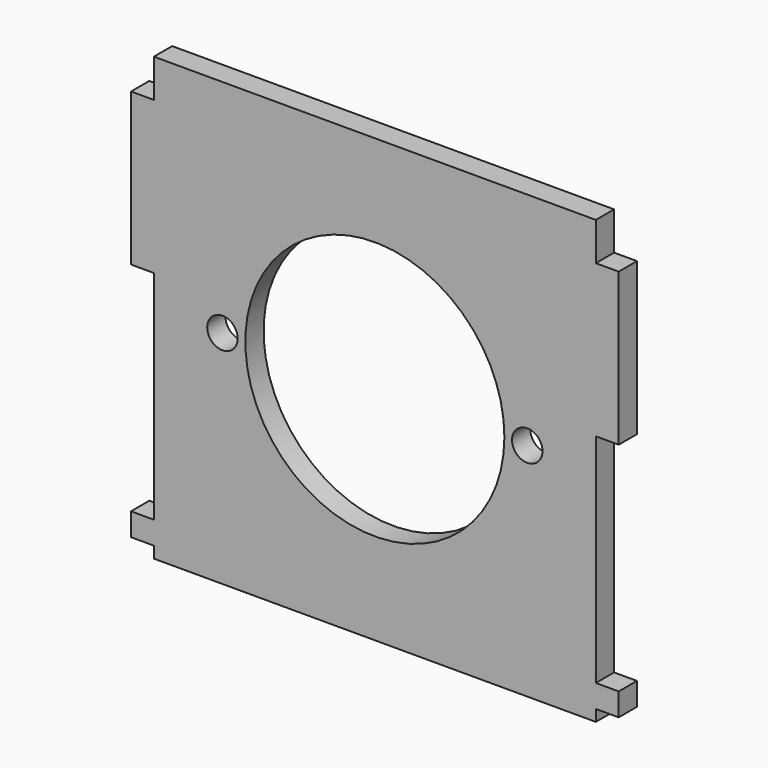
from build123d import *

# Parameters (mm, degrees)
F0_W     = 29
F0_H     = 29
F1_DEPTH = 1.5
F2_R     = 8.5
F3_DEPTH = 1.501
F4_R     = 1
F5_DEPTH = 1.501
F6_W     = 1.5
F6_H     = 1.5
F6_H_2   = 10
F7_DEPTH = 1.5


# Not quite as in the source:
# - a pattern or mirror of a feature is missing from the dataset's text; its kind, count and spacing are read off the source's solid


with BuildPart() as f1:
    # F0 (on Front) → F1 (new body)
    with BuildSketch(Plane.XZ):
        Rectangle(F0_W, F0_H)
    extrude(amount=F1_DEPTH)

    # F2 (on face) → F3 (cut, through all)
    with BuildSketch(Plane.XZ.offset(1.5)):
        Circle(F2_R)
    extrude(amount=-F3_DEPTH, mode=Mode.SUBTRACT)

    # F4 (on face) → F5 (cut, through all)
    with BuildSketch(Plane.XZ.offset(1.5)):
        with Locations((-10, 0)):
            Circle(F4_R)
    f5 = extrude(amount=-F5_DEPTH, mode=Mode.SUBTRACT)

    # F5_copies: F5 across plane
    add(f5.mirror(Plane(origin=(0, 0, 0), x_dir=(0, 0, 1), z_dir=(1, 0, 0))), mode=Mode.SUBTRACT)

    # F6 (on face) → F7 (join)
    with BuildSketch(Plane.XZ.offset(1.5)):
        with Locations((-15.25, -13)):
            Rectangle(F6_W, F6_H)
        with Locations((-15.25, 7)):
            Rectangle(F6_W, F6_H_2)
    f7 = extrude(amount=-F7_DEPTH)

    # F7_copies: F7 across plane
    add(f7.mirror(Plane(origin=(0, 0, 0), x_dir=(0, 0, 1), z_dir=(1, 0, 0))))


solid = f1.part
